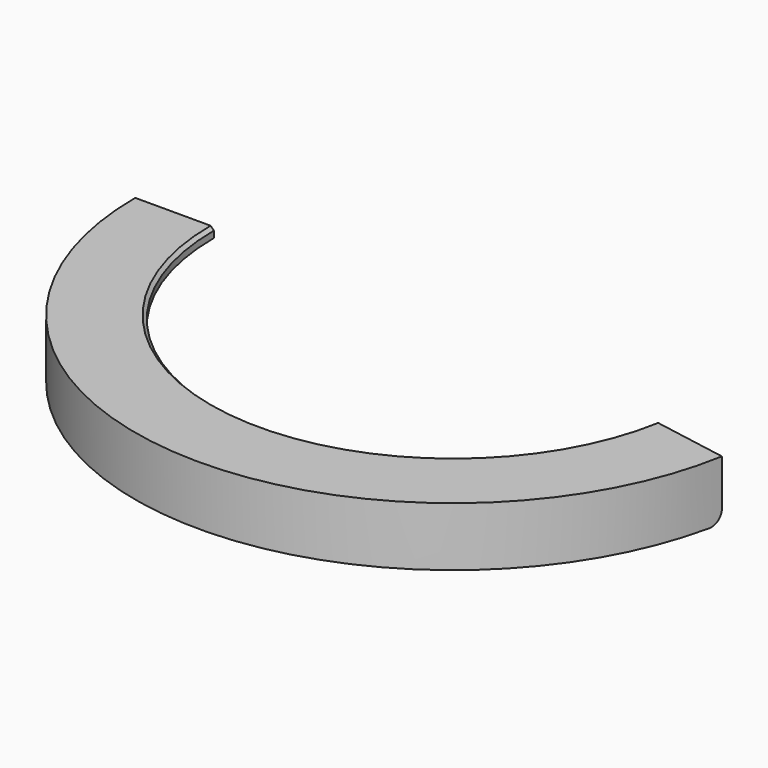
from build123d import *

# Parameters (mm, degrees)
F1_ANGLE = 170
F2_SIZE  = 0.5
F3_R     = 2
F4_SIZE  = 0.5


# Not quite as in the source:
# - a feature names something its author has since deleted; it is built from what else it names


with BuildPart() as f1:
    # F0 (on Front) → F1 (revolve)
    with BuildSketch(Plane.XZ):
        Polygon((-48.5, 9), (-48.5, 0), (-46.5, 0), (-46.5, 8), (-42.5, 8), (-38.5, 7.5), (-36.5, 7.5), (-36.5, 9), align=None)
    revolve(axis=Axis((0, 0, 4.2486875318), (0, 0, 1)), revolution_arc=F1_ANGLE)

    # F2
    f2_edges = [f1.edges().sort_by_distance(p)[0] for p in [
        (-4.052742, -46.323053, 0),
    ]]
    chamfer(f2_edges, length=F2_SIZE)

    # F3
    f3_edges = [f1.edges().sort_by_distance(p)[0] for p in [
        (47.02457, -8.2917, 0),
        (-47.75, 0, 0),
    ]]
    fillet(f3_edges, radius=F3_R)

    # F4
    f4_edges = [f1.edges().sort_by_distance(p)[0] for p in [
        (-3.181185, -36.361106, 9),
    ]]
    chamfer(f4_edges, length=F4_SIZE)


solid = f1.part
